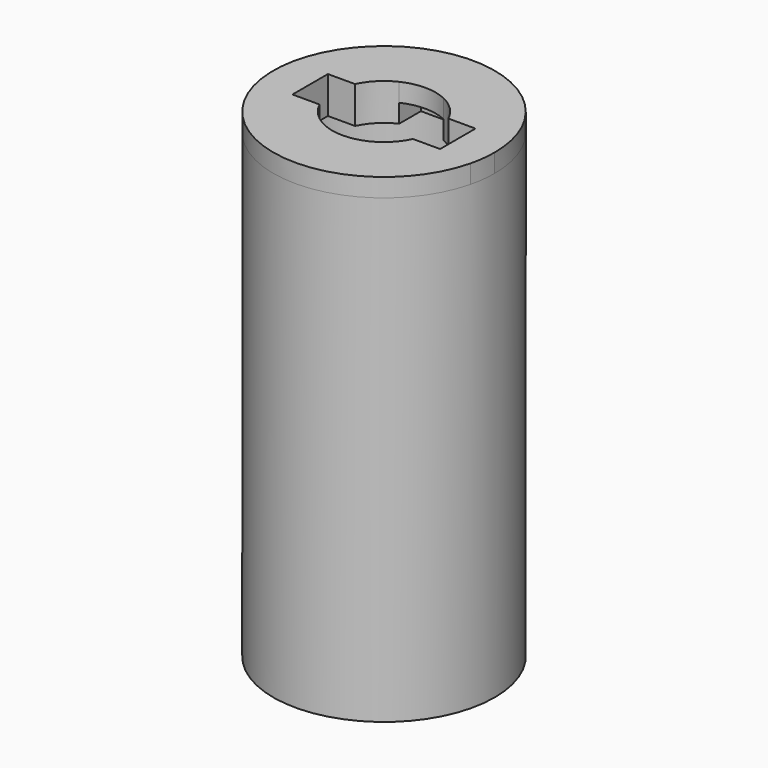
from build123d import *
from build123d import SkipClean  # not in build123d's __all__

# Parameters (mm, degrees)
F1_DEPTH  = 2.5
F3_DEPTH  = 2.5
F6_ANGLE  = 90
F8_R      = 12.5
F9_DEPTH  = 2.5
F10_DEPTH = 2.5
F13_DEPTH = 2.5


with BuildPart() as f1:
    # F0 (on Front) → F1 (new body)
    with BuildSketch(Plane.XZ):
        with BuildLine():
            ThreePointArc((-66.598045975, 33.1235192716), (-51.598045975, 18.1235192716), (-36.598045975, 33.1235192716))
            ThreePointArc((-36.598045975, 33.1235192716), (-51.598045975, 48.1235192716), (-66.598045975, 33.1235192716))
        make_face()
        with BuildLine():
            ThreePointArc((-48.598045975, 39.4480745919), (-46.6482985067, 38.0732667399), (-45.2734906546, 36.1235192716))
            Line((-45.2734906546, 36.1235192716), (-41.598045975, 36.1235192716))
            Line((-41.598045975, 36.1235192716), (-41.598045975, 30.1235192716))
            Line((-41.598045975, 30.1235192716), (-45.2734906546, 30.1235192716))
            ThreePointArc((-45.2734906546, 30.1235192716), (-46.6482985067, 28.1737718033), (-48.598045975, 26.7989639513))
            Line((-48.598045975, 26.7989639513), (-48.598045975, 23.1235192716))
            Line((-48.598045975, 23.1235192716), (-54.598045975, 23.1235192716))
            Line((-54.598045975, 23.1235192716), (-54.598045975, 26.7989639513))
            ThreePointArc((-54.598045975, 26.7989639513), (-56.5477934433, 28.1737718033), (-57.9226012953, 30.1235192716))
            Line((-57.9226012953, 30.1235192716), (-61.598045975, 30.1235192716))
            Line((-61.598045975, 30.1235192716), (-61.598045975, 36.1235192716))
            Line((-61.598045975, 36.1235192716), (-57.9226012953, 36.1235192716))
            ThreePointArc((-57.9226012953, 36.1235192716), (-56.5477934433, 38.0732667399), (-54.598045975, 39.4480745919))
            Line((-54.598045975, 39.4480745919), (-54.598045975, 43.1235192716))
            Line((-54.598045975, 43.1235192716), (-48.598045975, 43.1235192716))
            Line((-48.598045975, 43.1235192716), (-48.598045975, 39.4480745919))
        make_face(mode=Mode.SUBTRACT)
    extrude(amount=F1_DEPTH)

    # F2 (on face) → F3 (join)
    with BuildSketch(Plane(origin=(0, 0, 0), x_dir=(-1, 0, 0), z_dir=(0, 1, 0))):
        with BuildLine():
            ThreePointArc((66.598045975, 33.1235192716), (66.0446186482, 37.1604163471), (64.4251742419, 40.899429535))
            ThreePointArc((64.4251742419, 40.899429535), (36.7710486733, 30.8519226932), (66.164820243, 29.5445407268))
            ThreePointArc((66.164820243, 29.5445407268), (66.4893456835, 31.3209674721), (66.598045975, 33.1235192716))
        make_face()
        with BuildLine():
            ThreePointArc((54.598045975, 39.4480745919), (56.5477934433, 38.0732667399), (57.9226012953, 36.1235192716))
            Line((57.9226012953, 36.1235192716), (61.598045975, 36.1235192716))
            Line((61.598045975, 36.1235192716), (61.598045975, 30.1235192716))
            Line((61.598045975, 30.1235192716), (57.9226012953, 30.1235192716))
            ThreePointArc((57.9226012953, 30.1235192716), (56.5477934433, 28.1737718033), (54.598045975, 26.7989639513))
            ThreePointArc((54.598045975, 26.7989639513), (51.598045975, 26.1235192716), (48.598045975, 26.7989639513))
            ThreePointArc((48.598045975, 26.7989639513), (46.6482985067, 28.1737718033), (45.2734906546, 30.1235192716))
            Line((45.2734906546, 30.1235192716), (41.598045975, 30.1235192716))
            Line((41.598045975, 30.1235192716), (41.598045975, 36.1235192716))
            Line((41.598045975, 36.1235192716), (45.2734906546, 36.1235192716))
            ThreePointArc((45.2734906546, 36.1235192716), (46.6482985067, 38.0732667399), (48.598045975, 39.4480745919))
            ThreePointArc((48.598045975, 39.4480745919), (51.598045975, 40.1235192716), (54.598045975, 39.4480745919))
        make_face(mode=Mode.SUBTRACT)
    with SkipClean():  # cleaning this boolean's faces spoils the solid; the shape is the same uncleaned
        extrude(amount=F3_DEPTH)


with BuildPart() as f5:
    # F4 (on Front) → F5 (revolve)
    with BuildSketch(Plane.XZ):
        Polygon((6.781338717, -22.533902707), (6.781338717, 37.466097293), (4.281338717, 37.466097293), (4.281338717, 7.466097293), (-3.218661283, 7.466097293), (-3.218661283, 2.466097293), (0.8746451318, -17.533902707), (-4.1253548682, -17.533902707), (-4.218661283, -22.533902707), align=None)
    revolve(axis=Axis((-8.218661283, 0, -12.1948756373), (0, 0, -1)))

    # F8 (on offset) → F9 (join)
    with BuildSketch(Plane.XY.offset(37.466097293)):
        with BuildLine():
            ThreePointArc((-23.218661283, 0), (-8.218661283, -15), (6.781338717, 0))
            ThreePointArc((6.781338717, 0), (-8.218661283, 15), (-23.218661283, 0))
        make_face()
        with Locations((-8.218661283, 0)):
            Circle(F8_R, mode=Mode.SUBTRACT)
    extrude(amount=F9_DEPTH)

    # F8 (on offset) → F10 (join)
    with BuildSketch(Plane.XY.offset(37.466097293)):
        with Locations((-8.218661283, 0)):
            Circle(F8_R)
        with BuildLine():
            ThreePointArc((-5.218661283, 6.3245553203), (-3.2689138147, 4.9497474683), (-1.8941059626, 3))
            Line((-1.8941059626, 3), (1.781338717, 3))
            Line((1.781338717, 3), (1.781338717, -3))
            Line((1.781338717, -3), (-1.8941059626, -3))
            ThreePointArc((-1.8941059626, -3), (-3.2689138147, -4.9497474683), (-5.218661283, -6.3245553203))
            Line((-5.218661283, -6.3245553203), (-5.218661283, -10))
            Line((-5.218661283, -10), (-11.218661283, -10))
            Line((-11.218661283, -10), (-11.218661283, -6.3245553203))
            ThreePointArc((-11.218661283, -6.3245553203), (-13.1684087513, -4.9497474683), (-14.5432166033, -3))
            Line((-14.5432166033, -3), (-18.218661283, -3))
            Line((-18.218661283, -3), (-18.218661283, 3))
            Line((-18.218661283, 3), (-14.5432166033, 3))
            ThreePointArc((-14.5432166033, 3), (-13.1684087513, 4.9497474683), (-11.218661283, 6.3245553203))
            Line((-11.218661283, 6.3245553203), (-11.218661283, 10))
            Line((-11.218661283, 10), (-5.218661283, 10))
            Line((-5.218661283, 10), (-5.218661283, 6.3245553203))
        make_face(mode=Mode.SUBTRACT)
    extrude(amount=F10_DEPTH)

    # F12 (on offset) → F13 (join)
    with BuildSketch(Plane.XY.offset(42.466097293)):
        with BuildLine():
            ThreePointArc((6.781338717, 0), (6.2279113902, 4.0368970755), (4.6084669839, 7.7759102634))
            ThreePointArc((4.6084669839, 7.7759102634), (-23.0456585847, -2.2715965784), (6.3481129851, -3.5789785448))
            ThreePointArc((6.3481129851, -3.5789785448), (6.6726384256, -1.8025517995), (6.781338717, 0))
        make_face()
        with BuildLine():
            ThreePointArc((-5.218661283, 6.3245553203), (-3.2689138147, 4.9497474683), (-1.8941059626, 3))
            Line((-1.8941059626, 3), (1.781338717, 3))
            Line((1.781338717, 3), (1.781338717, -3))
            Line((1.781338717, -3), (-1.8941059626, -3))
            ThreePointArc((-1.8941059626, -3), (-3.2689138147, -4.9497474683), (-5.218661283, -6.3245553203))
            ThreePointArc((-5.218661283, -6.3245553203), (-8.218661283, -7), (-11.218661283, -6.3245553203))
            ThreePointArc((-11.218661283, -6.3245553203), (-13.1684087513, -4.9497474683), (-14.5432166033, -3))
            Line((-14.5432166033, -3), (-18.218661283, -3))
            Line((-18.218661283, -3), (-18.218661283, 3))
            Line((-18.218661283, 3), (-14.5432166033, 3))
            ThreePointArc((-14.5432166033, 3), (-13.1684087513, 4.9497474683), (-11.218661283, 6.3245553203))
            ThreePointArc((-11.218661283, 6.3245553203), (-8.218661283, 7), (-5.218661283, 6.3245553203))
        make_face(mode=Mode.SUBTRACT)
    extrude(amount=-F13_DEPTH)


with BuildPart() as f1_1:
    # F6: moved
    add(f1.part.rotate(Axis((-43.4357683148, 2.5, 36.1235192716), (-1, 0, 0)), F6_ANGLE), clean=False)


solid = f5.part
